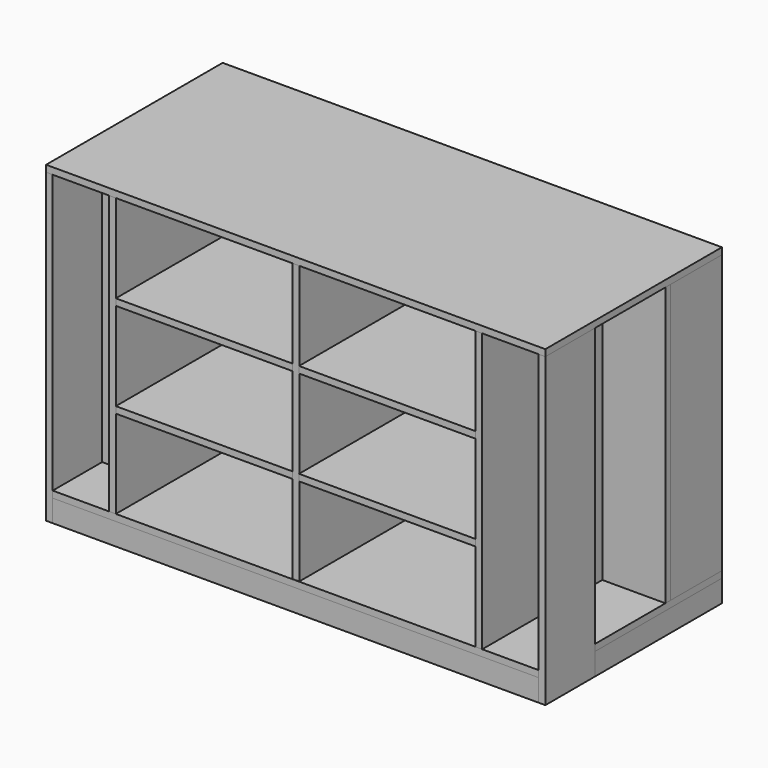
from build123d import *

# Parameters (mm, degrees)
F0_W      = 500
F0_H      = 695
F1_DEPTH  = 15
F2_W      = 1131
F2_H      = 500
F3_DEPTH  = 15
F4_W      = 500
F4_H      = 15
F5_DEPTH  = 1101
F6_W      = 15
F6_H      = 485
F7_DEPTH  = 50
F8_W      = 1101
F8_H      = 50
F9_DEPTH  = 15
F10_W     = 140
F10_H     = 695
F11_DEPTH = 15
F12_W     = 360
F12_H     = 15
F13_DEPTH = 15
F14_W     = 15
F14_H     = 360
F15_DEPTH = 50
F16_W     = 15
F16_H     = 500
F17_DEPTH = 630
F18_W     = 350
F18_H     = 15
F19_DEPTH = 400
F20_W     = 350
F20_H     = 15
F21_DEPTH = 400
F22_W     = 815
F22_H     = 630
F23_DEPTH = 15
F24_W     = 500
F24_H     = 630
F25_DEPTH = 15
F26_W     = 400
F26_H     = 15
F27_DEPTH = 350
F29_W     = 350
F29_H     = 15
F30_DEPTH = 400
F31_W     = 350
F31_H     = 630
F32_DEPTH = 15
F33_W     = 15
F33_H     = 630
F34_DEPTH = 143
F35_W     = 128
F35_H     = 630
F36_DEPTH = 15
F37_W     = 15
F37_H     = 630
F38_DEPTH = 128
F39_W     = 15
F39_H     = 630
F40_DEPTH = 128
F41_W     = 15
F41_H     = 630
F42_DEPTH = 145


with BuildPart() as f1:
    # F0 (on Right) → F1 (new body)
    with BuildSketch(Plane.YZ):
        with Locations((-250, 347.5)):
            Rectangle(F0_W, F0_H)
    extrude(amount=F1_DEPTH)


with BuildPart() as f3:
    # F2 (on face) → F3 (new body)
    with BuildSketch(Plane.XY.offset(695)):
        with Locations((565.5, -250)):
            Rectangle(F2_W, F2_H)
    extrude(amount=F3_DEPTH)


with BuildPart() as f5:
    # F4 (on face) → F5 (new body)
    with BuildSketch(Plane.YZ.offset(15)):
        with Locations((-250, 57.5)):
            Rectangle(F4_W, F4_H)
    extrude(amount=F5_DEPTH)

    # F12 (on face) → F13 (join)
    with BuildSketch(Plane.YZ.offset(1116)):
        with Locations((-180, 57.5)):
            Rectangle(F12_W, F12_H)
    extrude(amount=F13_DEPTH)


with BuildPart() as f7:
    # F6 (on face) → F7 (new body)
    with BuildSketch(Plane(origin=(0, 0, 50), x_dir=(1, 0, 0), z_dir=(0, 0, -1))):
        with Locations((580.5, 242.5)):
            Rectangle(F6_W, F6_H)
    extrude(amount=F7_DEPTH)


with BuildPart() as f9:
    # F8 (on face) → F9 (new body)
    with BuildSketch(Plane.XZ.offset(485)):
        with Locations((565.5, 25)):
            Rectangle(F8_W, F8_H)
    extrude(amount=F9_DEPTH)


with BuildPart() as f11:
    # F10 (on face) → F11 (new body)
    with BuildSketch(Plane.YZ.offset(1116)):
        with Locations((-430, 347.5)):
            Rectangle(F10_W, F10_H)
    extrude(amount=F11_DEPTH)


with BuildPart() as f15:
    # F14 (on face) → F15 (new body)
    with BuildSketch(Plane(origin=(0, 0, 50), x_dir=(1, 0, 0), z_dir=(0, 0, -1))):
        with Locations((1123.5, 180)):
            Rectangle(F14_W, F14_H)
    extrude(amount=F15_DEPTH)


with BuildPart() as f17:
    # F16 (on face) → F17 (new body)
    with BuildSketch(Plane(origin=(0, 0, 695), x_dir=(1, 0, 0), z_dir=(0, 0, -1))):
        with Locations((150.5, 250)):
            Rectangle(F16_W, F16_H)
    extrude(amount=F17_DEPTH)


with BuildPart() as f19:
    # F18 (on face) → F19 (new body)
    with BuildSketch(Plane.YZ.offset(158)):
        with Locations((-325, 487.5)):
            Rectangle(F18_W, F18_H)
    extrude(amount=F19_DEPTH)


with BuildPart() as f21:
    # F20 (on face) → F21 (new body)
    with BuildSketch(Plane.YZ.offset(158)):
        with Locations((-325, 272.5)):
            Rectangle(F20_W, F20_H)
    extrude(amount=F21_DEPTH)


with BuildPart() as f23:
    # F22 (on face) → F23 (new body)
    with BuildSketch(Plane(origin=(0, -150, 0), x_dir=(-1, 0, 0), z_dir=(0, 1, 0))):
        with Locations((-565.5, 380)):
            Rectangle(F22_W, F22_H)
    extrude(amount=F23_DEPTH)


with BuildPart() as f25:
    # F24 (on face) → F25 (new body)
    with BuildSketch(Plane.YZ.offset(973)):
        with Locations((-250, 380)):
            Rectangle(F24_W, F24_H)
    extrude(amount=F25_DEPTH)


with BuildPart() as f27:
    # F26 (on face) → F27 (new body)
    with BuildSketch(Plane.XZ.offset(150)):
        with Locations((773, 272.5)):
            Rectangle(F26_W, F26_H)
    extrude(amount=F27_DEPTH)


with BuildPart() as f30:
    # F29 (on face) → F30 (new body)
    with BuildSketch(Plane(origin=(973, 0, 0), x_dir=(0, -1, 0), z_dir=(-1, 0, 0))):
        with Locations((325, 487.5)):
            Rectangle(F29_W, F29_H)
    extrude(amount=F30_DEPTH)


with BuildPart() as f32:
    # F31 (on face) → F32 (new body)
    with BuildSketch(Plane.YZ.offset(558)):
        with Locations((-324.248115566, 380)):
            Rectangle(F31_W, F31_H)
    extrude(amount=F32_DEPTH)


with BuildPart() as f34:
    # F33 (on face) → F34 (new body)
    with BuildSketch(Plane.YZ.offset(988)):
        with Locations((-152.5, 380)):
            Rectangle(F33_W, F33_H)
    extrude(amount=F34_DEPTH)


with BuildPart() as f36:
    # F35 (on Front) → F36 (new body)
    with BuildSketch(Plane.XZ):
        with Locations((79, 380)):
            Rectangle(F35_W, F35_H)
    extrude(amount=F36_DEPTH)


with BuildPart() as f38:
    # F37 (on face) → F38 (new body)
    with BuildSketch(Plane.YZ.offset(15)):
        with Locations((-352.5, 380)):
            Rectangle(F37_W, F37_H)
    extrude(amount=F38_DEPTH)


with BuildPart() as f40:
    # F39 (on face) → F40 (new body)
    with BuildSketch(Plane.YZ.offset(988)):
        with Locations((-7.5, 380)):
            Rectangle(F39_W, F39_H)
    extrude(amount=F40_DEPTH)


with BuildPart() as f42:
    # F41 (on face) → F42 (new body)
    with BuildSketch(Plane(origin=(0, -145, 0), x_dir=(-1, 0, 0), z_dir=(0, 1, 0))):
        with Locations((-1123.5, 380)):
            Rectangle(F41_W, F41_H)
    extrude(amount=F42_DEPTH)


solid = Compound([f1.part, f3.part, f5.part, f7.part, f9.part, f11.part, f15.part, f17.part, f19.part, f21.part, f23.part, f25.part, f27.part, f30.part, f32.part, f34.part, f36.part, f38.part, f40.part, f42.part])
